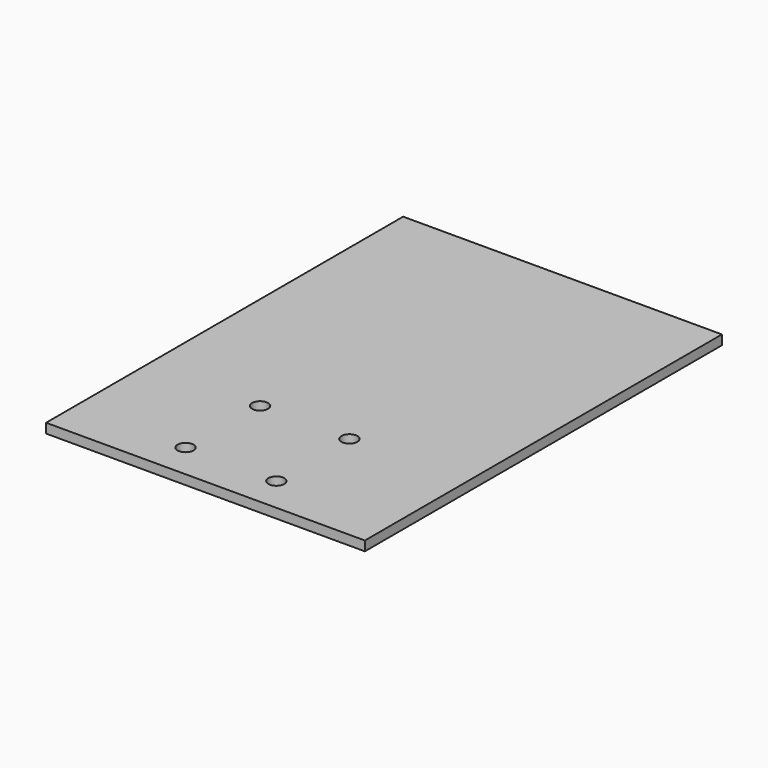
from build123d import *

# Parameters (mm, degrees)
F1_W     = 100
F1_H     = 140
F2_DEPTH = 3
F7_D     = 5


# Not quite as in the source:
# - the program builds the solid bodies; features that only make, move or delete a surface that nothing else refers to are left out


with BuildPart() as f2:
    # F1 (on face) → F2 (new body)
    with BuildSketch(Plane.XY):
        with Locations((50, -29.3391620165)):
            Rectangle(F1_W, F1_H)
    extrude(amount=F2_DEPTH)

    # F7 (through all)
    with Locations(Plane.XY.offset(3)):
        with Locations((35.3542789817, -59.622079134), (34.9003225565, -88.2757753134), (63.376352191, -59.622079134), (63.376352191, -88.2757753134)):
            Hole(F7_D / 2)


solid = f2.part
